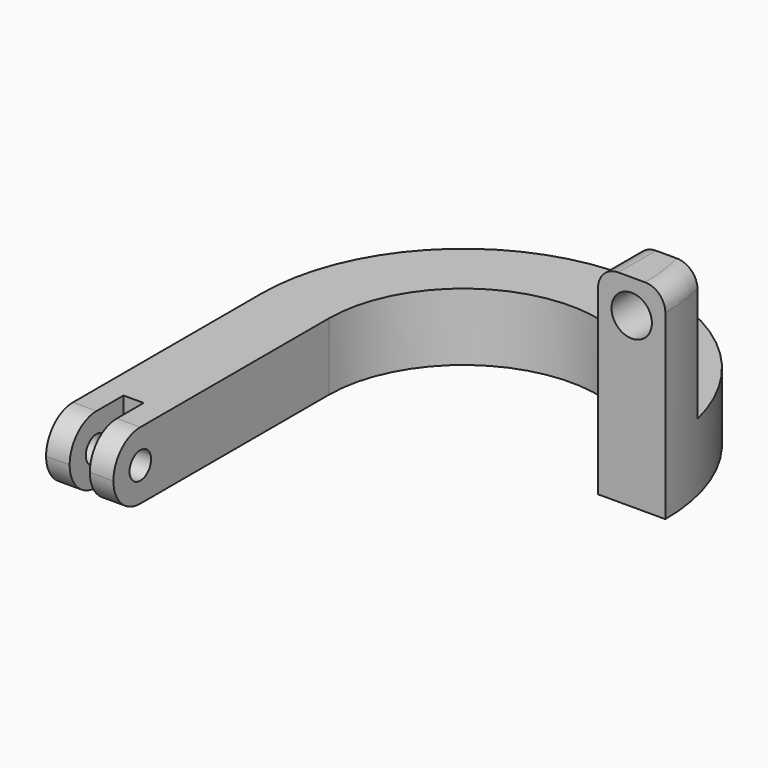
from build123d import *

# Parameters (mm, degrees)
F1_DEPTH = 10
F2_R     = 4.99999
F3_R     = 2
F4_DEPTH = 25
F6_DEPTH = 30
F7_R     = 3
F8_R     = 3
F9_DEPTH = 25


# Not quite as in the source:
# - a fillet or chamfer is up to 0.001 mm smaller than in the source, because OpenCascade refuses the exact size


with BuildPart() as f1:
    # F0 (on Top) → F1 (new body)
    with BuildSketch(Plane.XY):
        with BuildLine():
            ThreePointArc((-20, 0), (0, 20), (20, 0))
            Line((20, 0), (30, 0))
            ThreePointArc((30, 0), (0, 30), (-30, 0))
            Line((-30, 0), (-30, -40))
            Line((-30, -40), (-26.5, -40))
            Line((-26.5, -40), (-26.5, -30))
            Line((-26.5, -30), (-23.5, -30))
            Line((-23.5, -30), (-23.5, -40))
            Line((-23.5, -40), (-20, -40))
            Line((-20, -40), (-20, 0))
        make_face()
    extrude(amount=F1_DEPTH)

    # F2 (radius 5 in the source; OpenCascade refuses exactly that, so slightly less here)
    f2_edges = [f1.edges().sort_by_distance(p)[0] for p in [
        (-28.25, -40, 10),
        (-28.25, -40, 0),
        (-21.75, -40, 10),
        (-21.75, -40, 0),
    ]]
    fillet(f2_edges, radius=F2_R)

    # F3 (on face) → F4 (cut)
    with BuildSketch(Plane.YZ.offset(-20)):
        with Locations((-35, 5)):
            Circle(F3_R)
    extrude(amount=-F4_DEPTH, mode=Mode.SUBTRACT)

    # F5 (on face) → F6 (join)
    with BuildSketch(Plane(origin=(0, 0, 0), x_dir=(1, 0, 0), z_dir=(0, 0, -1))):
        with BuildLine():
            ThreePointArc((29.1719042916, -7), (29.7922567855, -3.5244057124), (30, 0))
            Line((30, 0), (20, 0))
            Line((20, 0), (20, -7))
            Line((20, -7), (29.1719042916, -7))
        make_face()
    extrude(amount=-F6_DEPTH)

    # F7
    f7_edges = [f1.edges().sort_by_distance(p)[0] for p in [
        (29.792257, 3.524406, 30),
        (20, 3.5, 30),
    ]]
    fillet(f7_edges, radius=F7_R)

    # F8 (on face) → F9 (cut)
    with BuildSketch(Plane(origin=(0, 7, 0), x_dir=(-1, 0, 0), z_dir=(0, 1, 0))):
        with Locations((-25, 25)):
            Circle(F8_R)
    extrude(amount=-F9_DEPTH, mode=Mode.SUBTRACT)


solid = f1.part
